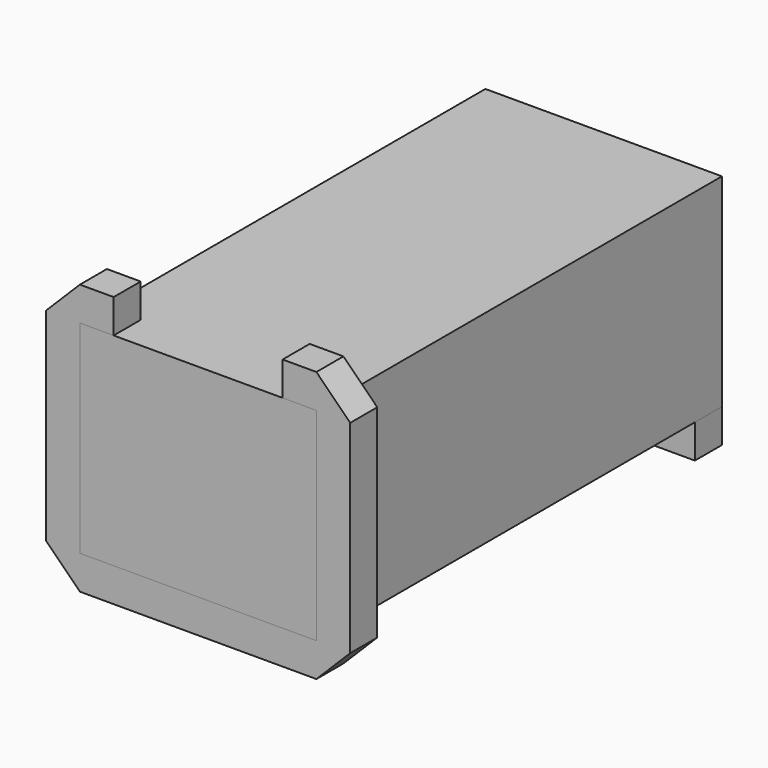
from build123d import *

# Parameters (mm, degrees)
F0_W     = 15
F0_H     = 32.5
F0_H_2   = 5
F0_W_2   = 5
F1_DEPTH = 30
F2_DEPTH = 5
F3_DEPTH = 35
F4_W     = 5
F4_H     = 5
F5_DEPTH = 5
F7_DEPTH = 5
F9_DEPTH = 75


# Not quite as in the source:
# - a feature names something its author has since deleted; it is built from what else it names


with BuildPart() as f1:
    # F0 (on Top) → F1 (new body)
    with BuildSketch(Plane.XY):
        Polygon((-2.5, 0), (0, 0), (2.5, 0), (2.5, 32.5), (-2.5, 32.5), align=None)
        with Locations((-10, 16.25)):
            Rectangle(F0_W, F0_H)
        Polygon((2.5, 0), (0, 0), (-2.5, 0), (-2.5, -32.5), (2.5, -32.5), align=None)
        with Locations((-10, -16.25)):
            Rectangle(F0_W, F0_H)
        with Locations((10, 16.25)):
            Rectangle(F0_W, F0_H)
        with Locations((10, -16.25)):
            Rectangle(F0_W, F0_H)
        Polygon((-2.5, 32.5), (2.5, 32.5), (2.5, 37.5), (0, 37.5), (-2.5, 37.5), align=None)
        with Locations((10, 35)):
            Rectangle(F0_W, F0_H_2)
        with Locations((-10, 35)):
            Rectangle(F0_W, F0_H_2)
        with Locations((10, -35)):
            Rectangle(F0_W, F0_H_2)
        with Locations((-10, -35)):
            Rectangle(F0_W, F0_H_2)
        with Locations((0, -35)):
            Rectangle(F0_W_2, F0_H_2)
    extrude(amount=F1_DEPTH)


with BuildPart() as f2:
    # F0 (on Top) → F2 (new body)
    with BuildSketch(Plane.XY):
        with Locations((-10, -35)):
            Rectangle(F0_W, F0_H_2)
        with Locations((-10, 35)):
            Rectangle(F0_W, F0_H_2)
        with Locations((10, -35)):
            Rectangle(F0_W, F0_H_2)
        Polygon((-2.5, 0), (0, 0), (2.5, 0), (2.5, 32.5), (-2.5, 32.5), align=None)
        with Locations((10, 35)):
            Rectangle(F0_W, F0_H_2)
        Polygon((-2.5, 32.5), (2.5, 32.5), (2.5, 37.5), (0, 37.5), (-2.5, 37.5), align=None)
        Polygon((2.5, 0), (0, 0), (-2.5, 0), (-2.5, -32.5), (2.5, -32.5), align=None)
        with Locations((0, -35)):
            Rectangle(F0_W_2, F0_H_2)
        with Locations((20, -35)):
            Rectangle(F0_W_2, F0_H_2)
        with Locations((-20, -35)):
            Rectangle(F0_W_2, F0_H_2)
    extrude(amount=-F2_DEPTH)

    # F0 (on Top) → F3 (join)
    with BuildSketch(Plane.XY):
        with Locations((-20, -35)):
            Rectangle(F0_W_2, F0_H_2)
        with Locations((20, -35)):
            Rectangle(F0_W_2, F0_H_2)
    extrude(amount=F3_DEPTH)

    # F4 (on face) → F5 (join)
    with BuildSketch(Plane.XZ.offset(37.5)):
        with Locations((-15, 32.5)):
            Rectangle(F4_W, F4_H)
        with Locations((15, 32.5)):
            Rectangle(F4_W, F4_H)
    extrude(amount=-F5_DEPTH)

    # F6 (on face) → F7 (cut)
    with BuildSketch(Plane(origin=(-2.5, 0, 0), x_dir=(0, -1, 0), z_dir=(-1, 0, 0))):
        Polygon((-30, -2.5), (-32.5, -5), (32.5, -5), (30, -2.5), align=None)
    extrude(amount=-F7_DEPTH, mode=Mode.SUBTRACT)

    # F8 (on face) → F9 (cut)
    with BuildSketch(Plane.XZ.offset(37.5)):
        Polygon((-22.5, 35), (-22.5, 30), (-17.5, 35), align=None)
        Polygon((17.5, 35), (22.5, 30), (22.5, 35), align=None)
        Polygon((-17.5, -5), (-22.5, 0), (-22.5, -5), align=None)
        Polygon((22.5, 0), (17.5, -5), (22.5, -5), align=None)
    extrude(amount=-F9_DEPTH, mode=Mode.SUBTRACT)


solid = Compound([f1.part, f2.part])
